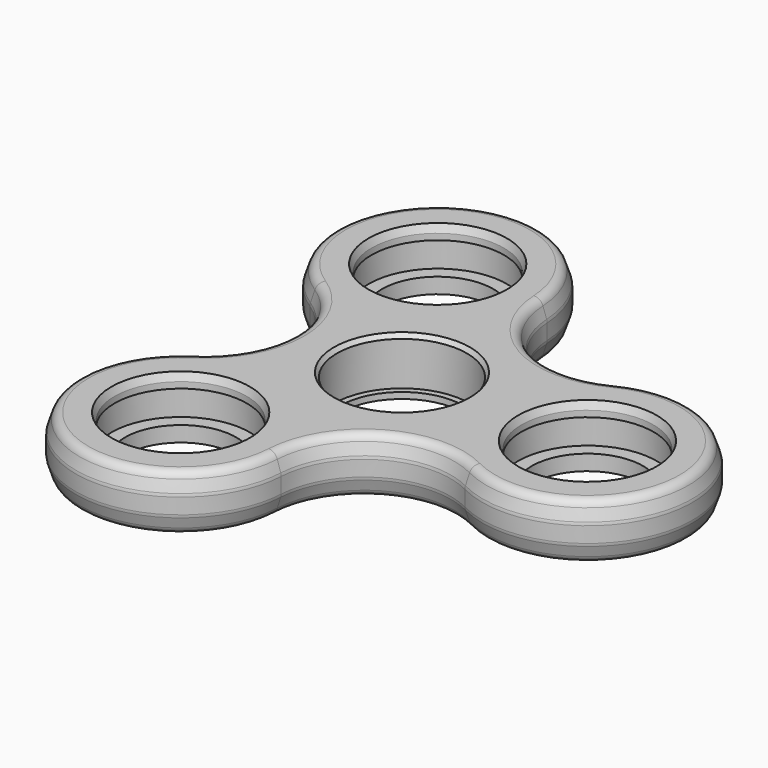
from build123d import *

# Parameters (mm, degrees)
F1_DEPTH        = 9
F5_COPIES_COUNT = 3
F6_SIZE2        = 1
F6_SIZE         = 3
F7_R            = 1.5


# Not quite as in the source:
# - a pattern or mirror of a feature is missing from the dataset's text; its kind, count and spacing are read off the source's solid


with BuildPart() as f1:
    # F0 (on Top) → F1 (new body)
    with BuildSketch(Plane.XY):
        with BuildLine():
            ThreePointArc((1.9757433376, -26.8885826556), (8.9557672626, -15.5118439197), (22.2983239827, -15.1553352495))
            ThreePointArc((22.2983239827, -15.1553352495), (47, 0), (22.2983239827, 15.1553352495))
            ThreePointArc((22.2983239827, 15.1553352495), (8.9557672626, 15.5118439197), (1.9757433376, 26.8885826556))
            ThreePointArc((1.9757433376, 26.8885826556), (-23.5, 40.7031939779), (-24.2740673203, 11.7332474061))
            ThreePointArc((-24.2740673203, 11.7332474061), (-17.9115345253, 0), (-24.2740673203, -11.7332474061))
            ThreePointArc((-24.2740673203, -11.7332474061), (-23.5, -40.7031939779), (1.9757433376, -26.8885826556))
        make_face()
    extrude(amount=F1_DEPTH)

    # F2 (on Right) → F3 (revolve, cut)
    with BuildSketch(Plane.YZ):
        Polygon((0, 9), (0, 0), (10, 0), (10, 1), (11, 1), (11, 8.3), (10.5, 8.3), (11, 9), align=None)
    revolve(axis=Axis((0, 0, 3.7751235068), (0, 0, -1)), mode=Mode.SUBTRACT)

    # F4 (on Front) → F5 (revolve, cut)
    with BuildSketch(Plane.XZ):
        Polygon((21, 0), (30, 0), (30, 9), (18.8, 9), (19.3, 7.8), (19.3, 6.8), (18.8, 6.8), (18.8, 2.5), (21, 2.5), align=None)
    f5 = revolve(axis=Axis((30, 0, 6.29213918), (0, 0, -1)), mode=Mode.SUBTRACT)

    # F5_copies: F5 ×3 about axis
    f5_copies_axis = Axis((0, 0, 0), (0, 0, 1))
    for i in range(1, F5_COPIES_COUNT):
        add(f5.rotate(f5_copies_axis, i * 360 / F5_COPIES_COUNT), mode=Mode.SUBTRACT)

    # F6
    f6_edges = [f1.edges().sort_by_distance(p)[0] for p in [
        (8.955767, -15.511844, 9),
        (8.955767, -15.511844, 0),
    ]]
    f6_side = f1.faces().sort_by_distance((8.955767, -15.511844, 4.5))[0]
    chamfer(f6_edges, length=F6_SIZE, length2=F6_SIZE2, reference=f6_side)

    # F7
    f7_edges = [f1.edges().sort_by_distance(p)[0] for p in [
        (8.455767, -14.645819, 9),
        (8.955767, -15.511844, 6),
        (8.955767, -15.511844, 3),
        (8.455767, -14.645819, 0),
        (-23.5, -40.703194, 3),
        (-23.5, -40.703194, 6),
        (-17.911535, 0, 3),
        (-17.911535, 0, 6),
        (-23, -39.837169, 0),
        (-23, -39.837169, 9),
        (-23.5, 40.703194, 3),
        (-23.5, 40.703194, 6),
        (-16.911535, 0, 0),
        (-16.911535, 0, 9),
        (46, 0, 0),
        (8.455767, 14.645819, 0),
        (-23, 39.837169, 0),
        (46, 0, 9),
        (8.455767, 14.645819, 9),
        (-23, 39.837169, 9),
        (47, 0, 3),
        (47, 0, 6),
        (8.955767, 15.511844, 3),
        (8.955767, 15.511844, 6),
    ]]
    fillet(f7_edges, radius=F7_R)


solid = f1.part
